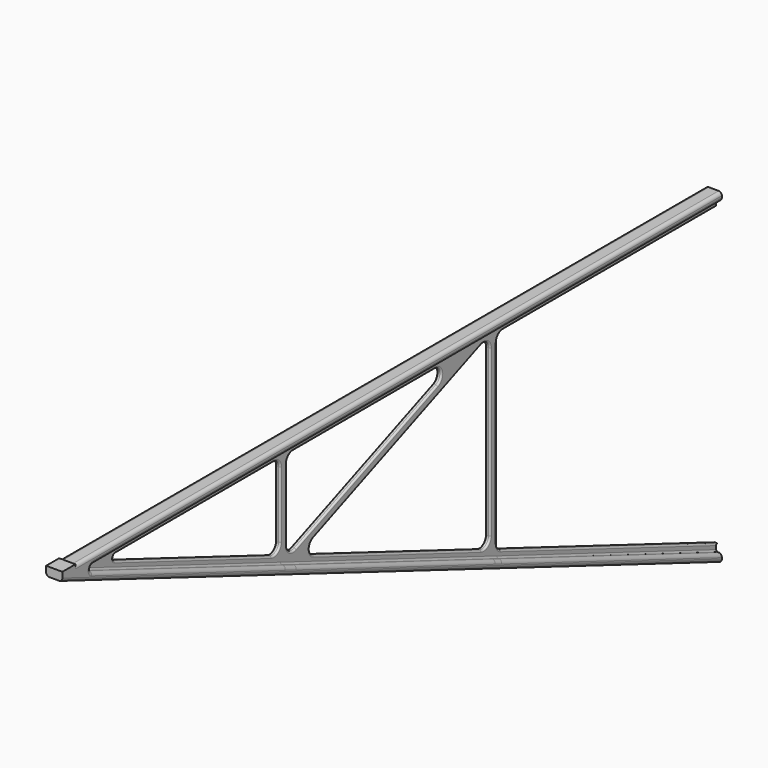
from build123d import *

# Parameters (mm, degrees)
F1_DEPTH  = 505
F2_DEPTH  = 500.5
F4_DEPTH  = 10
F5_DEPTH  = 10
F7_DEPTH  = 3.5
F8_W      = 10
F8_H      = 10
F10_DEPTH = 0.5
F11_DEPTH = 3.5
F12_W     = 3
F12_H     = 158.2
F12_H_2   = 149.0364306936
F12_H_3   = 168.1512820513
F13_DEPTH = 4
F14_W     = 3
F14_H     = 180.2518238002
F14_H_2   = 163.2489754916
F14_H_3   = 158.4799959846
F15_DEPTH = 4
F16_DEPTH = 40
F17_R     = 2
F18_R     = 5
F19_R     = 1
F20_R     = 2
F22_W     = 5.5675039161
F22_H     = 3.688506484
F23_DEPTH = 25


# Not quite as in the source:
# - two fillets or chamfers of one size are made in one step


with BuildPart() as f1:
    # F0 (on Front) → F1 (new body)
    with BuildSketch(Plane.XZ):
        Polygon((5, 0), (0, 0), (-5, 0), (-5, -200), (5, -200), align=None)
    extrude(amount=F1_DEPTH)

    # F0 (on Front) → F2 (join)
    with BuildSketch(Plane.XZ):
        Polygon((5, 0), (0, 0), (-5, 0), (-5, -200), (5, -200), align=None)
    extrude(amount=F2_DEPTH)

    # F3 (on face) → F4 (cut, through all)
    with BuildSketch(Plane(origin=(-5, 0, 0), x_dir=(0, -1, 0), z_dir=(-1, 0, 0))):
        Polygon((328.8512820513, -65.3208171387), (328.8512820513, -5), (179.8148513577, -5), align=None)
        Polygon((173.1512820513, -128.1396039604), (325.4411393395, -69.334609562), (173.1512820513, -7.6970046434), align=None)
        Polygon((168.1512820513, -5), (0, -5), (0, -195), (168.1512820513, -130.0702970297), align=None)
        Polygon((333.8512820513, -66.0871287129), (492.0512820513, -5), (333.8512820513, -5), align=None)
    extrude(amount=-F4_DEPTH, mode=Mode.SUBTRACT)

    # F3 (on face) → F5 (cut, through all)
    with BuildSketch(Plane(origin=(-5, 0, 0), x_dir=(0, -1, 0), z_dir=(-1, 0, 0))):
        Polygon((505, -200), (505, -5), (331.3512820513, -72.0524752475), (0, -200), align=None)
    extrude(amount=-F5_DEPTH, mode=Mode.SUBTRACT)

    # F6 (on face) → F7 (cut)
    with BuildSketch(Plane(origin=(-5, 0, 0), x_dir=(0, -1, 0), z_dir=(-1, 0, 0))):
        Polygon((179.8148513577, -5), (168.1512820513, -5), (168.1512820513, -130.0702970297), (173.1512820513, -128.1396039604), (173.1512820513, -7.6970046434), (325.4411393395, -69.334609562), (333.8512820513, -66.0871287129), (333.8512820513, -5), (328.8512820513, -5), (328.8512820513, -65.3208171387), align=None)
    extrude(amount=-F7_DEPTH, mode=Mode.SUBTRACT)

    # F8 (on face) → F10 (join)
    with BuildSketch(Plane.XY):
        with Locations((0, -500)):
            Rectangle(F8_W, F8_H)
    extrude(amount=F10_DEPTH)

    # F9 (on face) → F11 (cut)
    with BuildSketch(Plane.YZ.offset(5)):
        Polygon((-173.1512820513, -7.6970046434), (-173.1512820513, -128.1396039604), (-168.1512820513, -130.0702970297), (-168.1512820513, -5), (-179.8148513577, -5), (-328.8512820513, -65.3208171387), (-328.8512820513, -5), (-333.8512820513, -5), (-333.8512820513, -66.0871287129), (-325.4411393395, -69.334609562), align=None)
    extrude(amount=-F11_DEPTH, mode=Mode.SUBTRACT)

    # F12 (on face) → F13 (join)
    with BuildSketch(Plane(origin=(0, 0, -5), x_dir=(1, 0, 0), z_dir=(0, 0, -1))):
        with Locations((0, 412.9512820513)):
            Rectangle(F12_W, F12_H)
        with Locations((0, 254.3330667045)):
            Rectangle(F12_W, F12_H_2)
        with Locations((0, 84.0756410256)):
            Rectangle(F12_W, F12_H_3)
    extrude(amount=F13_DEPTH)

    # F14 (on face) → F15 (join)
    with BuildSketch(Plane(origin=(0, -65.5267872377, -169.6975772053), x_dir=(1, 0, 0), z_dir=(0, 0.3602166214, 0.9328686862))):
        with Locations((0, -19.8836707273)):
            Rectangle(F14_W, F14_H)
        with Locations((0, -196.9938815385)):
            Rectangle(F14_W, F14_H_2)
        with Locations((0, -366.8737226384)):
            Rectangle(F14_W, F14_H_3)
    extrude(amount=F15_DEPTH)

    # F16 (add): a face of the model
    f16_faces = [f1.faces().sort_by_distance(p)[0] for p in [
        (0, -167.4308488085, -128.2045596573),
    ]]
    extrude(f16_faces, amount=F16_DEPTH)

    # F17
    f17_edges = [f1.edges().sort_by_distance(p)[0] for p in [
        (0, -470.587878, -9),
        (-3.25, -492.051282, -5),
        (3.25, -492.051282, -5),
    ]]
    fillet(f17_edges, radius=F17_R)

    # F18
    f18_edges = [f1.edges().sort_by_distance(p)[0] for p in [
        (0, -333.851282, -9),
        (0, -328.851282, -9),
        (0, -328.851282, -65.320817),
        (0, -333.851282, -61.79928),
        (0, -189.69777, -9),
        (0, -173.151282, -7.697005),
        (0, -168.151282, -9),
        (0, -173.151282, -123.851755),
        (0, -320.019504, -67.140264),
        (0, -168.151282, -125.782448),
    ]]
    fillet(f18_edges, radius=F18_R)

    # F19
    f19_edges = [f1.edges().sort_by_distance(p)[0] for p in [
        (-1.5, -241.020007, -101.932869),
        (1.5, -240.65979, -5),
        (-1.5, -240.65979, -5),
        (-1.5, -483.285728, -6.633581),
        (1.5, -81.755749, -159.143099),
        (1.5, -167.274716, -125.181278),
        (1.5, -168.151282, -68.176665),
        (1.5, -241.020007, -101.932869),
        (1.5, -166.686816, -10.464466),
        (1.5, -483.285728, -6.633581),
        (1.5, -81.575641, -9),
        (1.5, -244.087811, -96.460422),
        (1.5, -175.323334, -120.684685),
        (1.5, -311.422012, -67.071118),
        (1.5, -173.151282, -65.837979),
        (1.5, -244.162599, -36.438036),
        (1.5, -175.356587, -10.968664),
        (1.5, -328.851282, -35.951557),
        (1.5, -326.645977, -62.049158),
        (1.5, -327.386816, -10.464466),
        (1.5, -267.739048, -40.586328),
        (1.5, -269.614919, -9),
        (1.5, -210.470713, -13.044452),
        (1.5, -399.353729, -9),
        (1.5, -335.315748, -10.464466),
        (1.5, -461.822324, -10.633581),
        (1.5, -333.851282, -34.254388),
        (1.5, -400.614487, -36.019428),
        (1.5, -336.023334, -58.63221),
        (-1.5, -81.755749, -159.143099),
        (-1.5, -167.274716, -125.181278),
        (-1.5, -168.151282, -68.176665),
        (-1.5, -166.686816, -10.464466),
        (-1.5, -81.575641, -9),
        (-1.5, -244.087811, -96.460422),
        (-1.5, -175.323334, -120.684685),
        (-1.5, -311.422012, -67.071118),
        (-1.5, -173.151282, -65.837979),
        (-1.5, -244.162599, -36.438036),
        (-1.5, -175.356587, -10.968664),
        (-1.5, -328.851282, -35.951557),
        (-1.5, -326.645977, -62.049158),
        (-1.5, -327.386816, -10.464466),
        (-1.5, -267.739048, -40.586328),
        (-1.5, -269.614919, -9),
        (-1.5, -210.470713, -13.044452),
        (-1.5, -399.353729, -9),
        (-1.5, -335.315748, -10.464466),
        (-1.5, -461.822324, -10.633581),
        (-1.5, -333.851282, -34.254388),
        (-1.5, -400.614487, -36.019428),
        (-1.5, -336.023334, -58.63221),
    ]]
    fillet(f19_edges, radius=F19_R)

    # F20
    f20_edges = [f1.edges().sort_by_distance(p)[0] for p in [
        (-5, -240.65979, -5),
        (-5, -247.5, 0),
        (5, -247.5, 0),
        (5, -240.65979, -5),
        (5, -252.5, -102.5),
        (-5, -252.5, -102.5),
        (5, -241.020007, -101.932869),
        (5, -483.285728, -6.633581),
        (-5, -241.020007, -101.932869),
        (-5, -483.285728, -6.633581),
    ]]
    fillet(f20_edges, radius=F20_R)

    # F22 (on face) → F23 (cut)
    with BuildSketch(Plane(origin=(0, 0, 0), x_dir=(-1, 0, 0), z_dir=(0, 1, 0))):
        with Locations((-0.283751958, -193.155746758)):
            Rectangle(F22_W, F22_H)
    extrude(amount=F23_DEPTH, mode=Mode.SUBTRACT)


solid = f1.part
